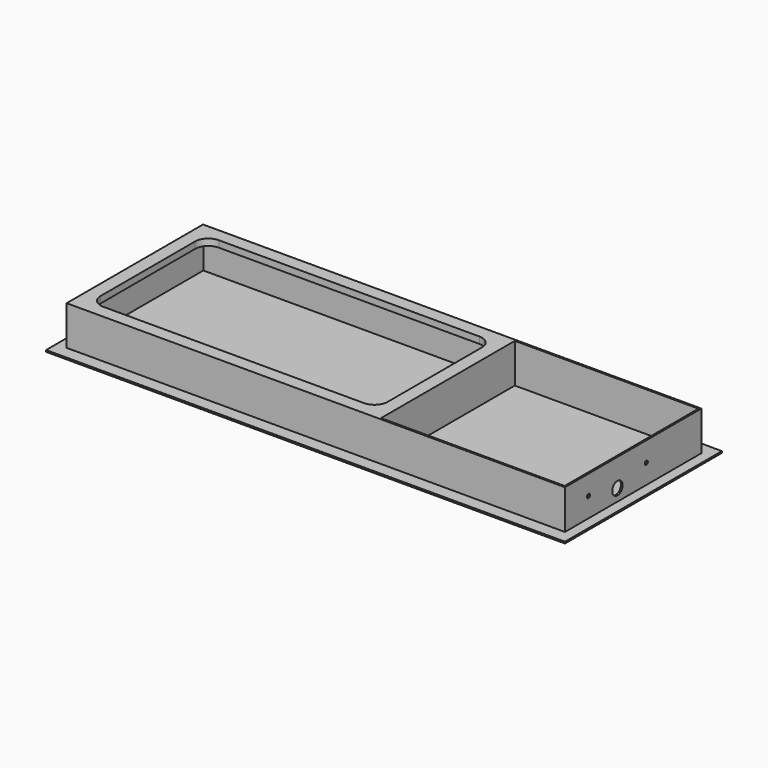
from build123d import *

# Parameters (mm, degrees)
F0_W        = 1005
F0_H        = 380
F1_DEPTH    = 3.175
F2_W        = 965.2
F2_H        = 330.2
F3_DEPTH    = 76.2
F4_T        = 3.175
F4_T3_DEPTH = 336.55
F4_T5_DEPTH = 971.55
F5_R        = 3.75
F5_R_2      = 12.5
F6_DEPTH    = 3.175
F7_W        = 3.175
F7_H        = 323.85
F8_DEPTH    = 63.5
F10_DEPTH   = 325
F12_DEPTH   = 12.7


# Not quite as in the source:
# - a shell that OpenCascade refuses in one call is made with other operations: the cavity is built on its own and cut out


with BuildPart() as f1:
    # F0 (on Top) → F1 (new body)
    with BuildSketch(Plane.XY):
        Rectangle(F0_W, F0_H)
    extrude(amount=-F1_DEPTH)

    # F2 (on face) → F3 (join)
    with BuildSketch(Plane.XY):
        Rectangle(F2_W, F2_H)
    extrude(amount=F3_DEPTH)

    # F4: shell of thickness 3.175, made by hand


with BuildPart() as f4_core1:
    # F4_t2: copy of F1
    add(f1.part)

    # the walls: a layer under each face that stays
    f4_faces = [f4_core1.faces().sort_by_distance(p)[0] for p in [
        (502.5, 0, -1.5875),
        (0, -190, -1.5875),
        (0, 190, -1.5875),
        (-469, -177.3333333333, 0),
        (0, 0, -3.175),
        (-502.5, 0, -1.5875),
        (482.6, 0, 38.1),
        (0, 165.1, 38.1),
        (-482.6, 0, 38.1),
        (0, -165.1, 38.1),
    ]]
    thicken(f4_faces, amount=-F4_T, mode=Mode.SUBTRACT)

    # F4_s4 → F4_t3 (cut)
    with BuildSketch(Plane.XZ.offset(-168.275)):
        Polygon((482.63175, 0.03175), (482.6, -3.175), (479.425, -3.175), (479.425, 0), align=None)
        Polygon((-482.63175, 0.03175), (-482.6, -3.175), (-479.425, -3.175), (-479.425, 0), align=None)
    extrude(amount=F4_T3_DEPTH, mode=Mode.SUBTRACT)

    # F4_s6 → F4_t5 (cut)
    with BuildSketch(Plane.YZ.offset(-485.775)):
        Polygon((165.13175, 0.03175), (165.1, -3.175), (161.925, -3.175), (161.925, 0), align=None)
        Polygon((-165.13175, 0.03175), (-165.1, -3.175), (-161.925, -3.175), (-161.925, 0), align=None)
    extrude(amount=F4_T5_DEPTH, mode=Mode.SUBTRACT)


with BuildPart() as f1_1:
    add(f1.part)

    # what is left inside the walls is the cavity
    f4_cavity = [f4_core1.part.solids().sort_by_distance(p)[0] for p in [
        (0, -53.975, 0.03175),
    ]]
    add(f4_cavity, mode=Mode.SUBTRACT)

    # F5 (on face) → F6 (cut)
    with BuildSketch(Plane.YZ.offset(482.6)):
        with Locations((-108.1, 38.1)):
            Circle(F5_R)
        with Locations((-38.1, 23.1)):
            Circle(F5_R_2)
        with Locations((31.9, 38.1)):
            Circle(F5_R)
    extrude(amount=-F6_DEPTH, mode=Mode.SUBTRACT)

    # F7 (on face) → F8 (join)
    with BuildSketch(Plane.XY):
        with Locations((122.2375, 0)):
            Rectangle(F7_W, F7_H)
    extrude(amount=F8_DEPTH)

    # F9 (on face) → F10 (join)
    with BuildSketch(Plane(origin=(0, -161.925, 0), x_dir=(-1, 0, 0), z_dir=(0, 1, 0))):
        Polygon((-123.825, 76.2), (-123.825, 63.5), (-120.65, 63.5), (479.425, 63.5), (479.425, 76.2), align=None)
    extrude(amount=F10_DEPTH)

    # F11 (on face) → F12 (cut)
    with BuildSketch(Plane.XY.offset(76.2)):
        with BuildLine():
            ThreePointArc((-457.2, -114.3), (-449.7605122421, -132.2605122421), (-431.8, -139.7))
            Line((-431.8, -139.7), (73.025, -139.7))
            ThreePointArc((73.025, -139.7), (90.9855122421, -132.2605122421), (98.425, -114.3))
            Line((98.425, -114.3), (98.425, 114.3))
            ThreePointArc((98.425, 114.3), (90.9855122421, 132.2605122421), (73.025, 139.7))
            Line((73.025, 139.7), (-431.8, 139.7))
            ThreePointArc((-431.8, 139.7), (-449.7605122421, 132.2605122421), (-457.2, 114.3))
            Line((-457.2, 114.3), (-457.2, -114.3))
        make_face()
    extrude(amount=-F12_DEPTH, mode=Mode.SUBTRACT)


solid = f1_1.part
